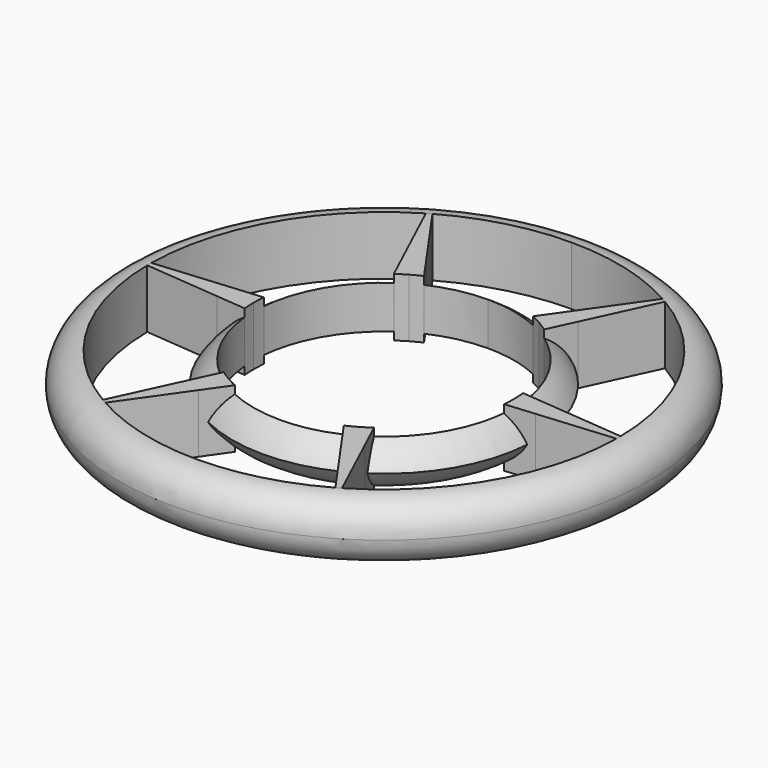
from build123d import *

# Parameters (mm, degrees)
F1_DEPTH      = 5
F3_T4_ANGLE   = 158.6510519463
F3_T9_ANGLE   = 158.6510519463
F3_T15_ANGLE  = 158.6510519463
F3_T20_ANGLE  = 158.6510519463
F3_T25_ANGLE  = 158.6510519463
F3_T31_ANGLE  = 158.6510519463
F3_T36_ANGLE  = 158.6510519463
F3_T41_ANGLE  = 158.6510519463
F3_T47_ANGLE  = 158.6510519463
F3_T52_ANGLE  = 158.6510519463
F3_T57_ANGLE  = 158.6510519463
F3_T63_ANGLE  = 158.6510519463
F3_T68_ANGLE  = 158.6510519463
F3_T73_ANGLE  = 158.6510519463
F3_T79_ANGLE  = 158.6510519463
F3_T84_ANGLE  = 158.6510519463
F3_T89_ANGLE  = 158.6510519463
F3_T95_ANGLE  = 158.6510519463
F3_T100_ANGLE = 158.6510519463
F3_T105_ANGLE = 158.6510519463
F3_T111_ANGLE = 158.6510519463
F3_T116_ANGLE = 158.6510519463
F3_T121_ANGLE = 158.6510519463
F3_T127_ANGLE = 158.6510519463
F3_T132_ANGLE = 158.6510519463
F3_T137_ANGLE = 158.6510519463
F3_T143_ANGLE = 158.6510519463
F3_T148_ANGLE = 158.6510519463
F3_T153_ANGLE = 158.6510519463
F3_T159_ANGLE = 158.6510519463
F3_T164_ANGLE = 158.6510519463
F3_T169_ANGLE = 158.6510519463
F3_T175_ANGLE = 158.6510519463
F3_T180_ANGLE = 158.6510519463
F3_T185_ANGLE = 158.6510519463
F3_T191_ANGLE = 158.6510519463


# Not quite as in the source:
# - a fillet or chamfer that OpenCascade refuses, or shapes differently, is made with other operations: its cross-section is extruded or revolved along the edge and cut away or added


with BuildPart() as f1:
    # F0 (on Top) → F1 (new body)
    with BuildSketch(Plane.XY):
        with BuildLine():
            Line((-6.4078035727, 9.0636666627), (-7.4753298331, 11.3613134754))
            ThreePointArc((-7.4753298331, 11.3613134754), (-11.7779454915, 6.8), (-13.5768510066, 0.7931687994))
            Line((-13.5768510066, 0.7931687994), (-11.0532673677, 1.0174873451))
            ThreePointArc((-11.0532673677, 1.0174873451), (-9.612881982, 5.55), (-6.4078035727, 9.0636666627))
        make_face()
        with BuildLine():
            Line((-11.0532673677, 1.0174873451), (-13.5768510066, 0.7931687994))
            ThreePointArc((-13.5768510066, 0.7931687994), (-13.5942115198, 0.3967532672), (-13.6, 0))
            Line((-13.6, 0), (-11.1, 0))
            ThreePointArc((-11.1, 0), (-11.088310687, 0.5092799909), (-11.0532673677, 1.0174873451))
        make_face()
        with BuildLine():
            ThreePointArc((-13.6, 0), (-13.5942115198, -0.3967532672), (-13.5768510066, -0.7931687994))
            Line((-13.5768510066, -0.7931687994), (-11.0532673677, -1.0174873451))
            ThreePointArc((-11.0532673677, -1.0174873451), (-11.088310687, -0.5092799909), (-11.1, 0))
            Line((-11.1, 0), (-13.6, 0))
        make_face()
        with BuildLine():
            ThreePointArc((-13.5768510066, -0.7931687994), (-11.7779454915, -6.8), (-7.4753298331, -11.3613134754))
            Line((-7.4753298331, -11.3613134754), (-6.4078035727, -9.0636666627))
            ThreePointArc((-6.4078035727, -9.0636666627), (-9.612881982, -5.55), (-11.0532673677, -1.0174873451))
            Line((-11.0532673677, -1.0174873451), (-13.5768510066, -0.7931687994))
        make_face()
        with BuildLine():
            Line((-6.4078035727, -9.0636666627), (-7.4753298331, -11.3613134754))
            ThreePointArc((-7.4753298331, -11.3613134754), (-7.1407041684, -11.5745558869), (-6.8, -11.7779454915))
            Line((-6.8, -11.7779454915), (-5.55, -9.612881982))
            ThreePointArc((-5.55, -9.612881982), (-5.9852047532, -9.3481187445), (-6.4078035727, -9.0636666627))
        make_face()
        with BuildLine():
            ThreePointArc((-6.8, -11.7779454915), (-6.4535073514, -11.9713091542), (-6.1015211735, -12.1544822748))
            Line((-6.1015211735, -12.1544822748), (-4.645463795, -10.0811540078))
            ThreePointArc((-4.645463795, -10.0811540078), (-5.1031059338, -9.8573987354), (-5.55, -9.612881982))
            Line((-5.55, -9.612881982), (-6.8, -11.7779454915))
        make_face()
        with BuildLine():
            ThreePointArc((0, -13.6), (3.135206617, -13.2336872968), (6.1015211735, -12.1544822748))
            Line((6.1015211735, -12.1544822748), (4.645463795, -10.0811540078))
            ThreePointArc((4.645463795, -10.0811540078), (2.3779392878, -10.8422970234), (0, -11.1))
            Line((0, -11.1), (0, -13.6))
        make_face()
        with BuildLine():
            Line((-4.645463795, -10.0811540078), (-6.1015211735, -12.1544822748))
            ThreePointArc((-6.1015211735, -12.1544822748), (-3.135206617, -13.2336872968), (0, -13.6))
            Line((0, -13.6), (0, -11.1))
            ThreePointArc((0, -11.1), (-2.3779392878, -10.8422970234), (-4.645463795, -10.0811540078))
        make_face()
        with BuildLine():
            Line((4.645463795, -10.0811540078), (6.1015211735, -12.1544822748))
            ThreePointArc((6.1015211735, -12.1544822748), (6.4535073514, -11.9713091542), (6.8, -11.7779454915))
            Line((6.8, -11.7779454915), (5.55, -9.612881982))
            ThreePointArc((5.55, -9.612881982), (5.1031059338, -9.8573987354), (4.645463795, -10.0811540078))
        make_face()
        with BuildLine():
            ThreePointArc((6.8, -11.7779454915), (7.1407041684, -11.5745558869), (7.4753298331, -11.3613134754))
            Line((7.4753298331, -11.3613134754), (6.4078035727, -9.0636666627))
            ThreePointArc((6.4078035727, -9.0636666627), (5.9852047532, -9.3481187445), (5.55, -9.612881982))
            Line((5.55, -9.612881982), (6.8, -11.7779454915))
        make_face()
        with BuildLine():
            ThreePointArc((7.4753298331, -11.3613134754), (11.7779454915, -6.8), (13.5768510066, -0.7931687994))
            Line((13.5768510066, -0.7931687994), (11.0532673677, -1.0174873451))
            ThreePointArc((11.0532673677, -1.0174873451), (9.612881982, -5.55), (6.4078035727, -9.0636666627))
            Line((6.4078035727, -9.0636666627), (7.4753298331, -11.3613134754))
        make_face()
        with BuildLine():
            ThreePointArc((13.5768510066, -0.7931687994), (13.5942115198, -0.3967532672), (13.6, 0))
            Line((13.6, 0), (11.1, 0))
            ThreePointArc((11.1, 0), (11.088310687, -0.5092799909), (11.0532673677, -1.0174873451))
            Line((11.0532673677, -1.0174873451), (13.5768510066, -0.7931687994))
        make_face()
        with BuildLine():
            Line((11.1, 0), (13.6, 0))
            ThreePointArc((13.6, 0), (13.5942115198, 0.3967532672), (13.5768510066, 0.7931687994))
            Line((13.5768510066, 0.7931687994), (11.0532673677, 1.0174873451))
            ThreePointArc((11.0532673677, 1.0174873451), (11.088310687, 0.5092799909), (11.1, 0))
        make_face()
        with BuildLine():
            Line((11.0532673677, 1.0174873451), (13.5768510066, 0.7931687994))
            ThreePointArc((13.5768510066, 0.7931687994), (11.7779454915, 6.8), (7.4753298331, 11.3613134754))
            Line((7.4753298331, 11.3613134754), (6.4078035727, 9.0636666627))
            ThreePointArc((6.4078035727, 9.0636666627), (9.612881982, 5.55), (11.0532673677, 1.0174873451))
        make_face()
        with BuildLine():
            Line((6.4078035727, 9.0636666627), (7.4753298331, 11.3613134754))
            ThreePointArc((7.4753298331, 11.3613134754), (7.1407041684, 11.5745558869), (6.8, 11.7779454915))
            Line((6.8, 11.7779454915), (5.55, 9.612881982))
            ThreePointArc((5.55, 9.612881982), (5.9852047532, 9.3481187445), (6.4078035727, 9.0636666627))
        make_face()
        with BuildLine():
            ThreePointArc((6.8, 11.7779454915), (6.4535073514, 11.9713091542), (6.1015211735, 12.1544822748))
            Line((6.1015211735, 12.1544822748), (4.645463795, 10.0811540078))
            ThreePointArc((4.645463795, 10.0811540078), (5.1031059338, 9.8573987354), (5.55, 9.612881982))
            Line((5.55, 9.612881982), (6.8, 11.7779454915))
        make_face()
        with BuildLine():
            Line((4.645463795, 10.0811540078), (6.1015211735, 12.1544822748))
            ThreePointArc((6.1015211735, 12.1544822748), (3.135206617, 13.2336872968), (0, 13.6))
            Line((0, 13.6), (0, 11.1))
            ThreePointArc((0, 11.1), (2.3779392878, 10.8422970234), (4.645463795, 10.0811540078))
        make_face()
        with BuildLine():
            ThreePointArc((0, 13.6), (-3.135206617, 13.2336872968), (-6.1015211735, 12.1544822748))
            Line((-6.1015211735, 12.1544822748), (-4.645463795, 10.0811540078))
            ThreePointArc((-4.645463795, 10.0811540078), (-2.3779392878, 10.8422970234), (0, 11.1))
            Line((0, 11.1), (0, 13.6))
        make_face()
        with BuildLine():
            Line((-4.645463795, 10.0811540078), (-6.1015211735, 12.1544822748))
            ThreePointArc((-6.1015211735, 12.1544822748), (-6.4535073514, 11.9713091542), (-6.8, 11.7779454915))
            Line((-6.8, 11.7779454915), (-5.55, 9.612881982))
            ThreePointArc((-5.55, 9.612881982), (-5.1031059338, 9.8573987354), (-4.645463795, 10.0811540078))
        make_face()
        with BuildLine():
            ThreePointArc((-6.8, 11.7779454915), (-7.1407041684, 11.5745558869), (-7.4753298331, 11.3613134754))
            Line((-7.4753298331, 11.3613134754), (-6.4078035727, 9.0636666627))
            ThreePointArc((-6.4078035727, 9.0636666627), (-5.9852047532, 9.3481187445), (-5.55, 9.612881982))
            Line((-5.55, 9.612881982), (-6.8, 11.7779454915))
        make_face()
        with BuildLine():
            Line((-10.1919273103, 17.2082717814), (-11.25, 19.4855715851))
            ThreePointArc((-11.25, 19.4855715851), (-19.4855715851, 11.25), (-22.5, 0))
            Line((-22.5, 0), (-19.998764173, 0.2223320735))
            ThreePointArc((-19.998764173, 0.2223320735), (-17.3205080757, 10), (-10.1919273103, 17.2082717814))
        make_face()
        with BuildLine():
            ThreePointArc((-22.5, 0), (-19.4855715851, -11.25), (-11.25, -19.4855715851))
            Line((-11.25, -19.4855715851), (-10.1919273103, -17.2082717814))
            ThreePointArc((-10.1919273103, -17.2082717814), (-17.3205080757, -10), (-19.998764173, -0.2223320735))
            Line((-19.998764173, -0.2223320735), (-22.5, 0))
        make_face()
        with BuildLine():
            ThreePointArc((-11.25, -19.4855715851), (0, -22.5), (11.25, -19.4855715851))
            Line((11.25, -19.4855715851), (9.8068368628, -17.4306038549))
            ThreePointArc((9.8068368628, -17.4306038549), (5.0689211328, -19.3469904261), (0, -20))
            ThreePointArc((0, -20), (-5.0689211328, -19.3469904261), (-9.8068368628, -17.4306038549))
            Line((-9.8068368628, -17.4306038549), (-11.25, -19.4855715851))
        make_face()
        with BuildLine():
            ThreePointArc((11.25, -19.4855715851), (19.4855715851, -11.25), (22.5, 0))
            Line((22.5, 0), (19.998764173, -0.2223320735))
            ThreePointArc((19.998764173, -0.2223320735), (17.3205080757, -10), (10.1919273103, -17.2082717814))
            Line((10.1919273103, -17.2082717814), (11.25, -19.4855715851))
        make_face()
        with BuildLine():
            Line((19.998764173, 0.2223320735), (22.5, 0))
            ThreePointArc((22.5, 0), (19.4855715851, 11.25), (11.25, 19.4855715851))
            Line((11.25, 19.4855715851), (10.1919273103, 17.2082717814))
            ThreePointArc((10.1919273103, 17.2082717814), (17.3205080757, 10), (19.998764173, 0.2223320735))
        make_face()
        with BuildLine():
            Line((9.8068368628, 17.4306038549), (11.25, 19.4855715851))
            ThreePointArc((11.25, 19.4855715851), (0, 22.5), (-11.25, 19.4855715851))
            Line((-11.25, 19.4855715851), (-9.8068368628, 17.4306038549))
            ThreePointArc((-9.8068368628, 17.4306038549), (-5.0689211328, 19.3469904261), (0, 20))
            ThreePointArc((0, 20), (5.0689211328, 19.3469904261), (9.8068368628, 17.4306038549))
        make_face()
        with BuildLine():
            Line((10.1919273103, 17.2082717814), (11.25, 19.4855715851))
            Line((11.25, 19.4855715851), (10, 17.3205080757))
            ThreePointArc((10, 17.3205080757), (10.0961196195, 17.2646566322), (10.1919273103, 17.2082717814))
        make_face()
        with BuildLine():
            Line((10, 17.3205080757), (11.25, 19.4855715851))
            Line((11.25, 19.4855715851), (9.8068368628, 17.4306038549))
            ThreePointArc((9.8068368628, 17.4306038549), (9.9035714213, 17.3758243863), (10, 17.3205080757))
        make_face()
        with BuildLine():
            Line((-9.8068368628, 17.4306038549), (-11.25, 19.4855715851))
            Line((-11.25, 19.4855715851), (-10, 17.3205080757))
            ThreePointArc((-10, 17.3205080757), (-9.9035714213, 17.3758243863), (-9.8068368628, 17.4306038549))
        make_face()
        with BuildLine():
            Line((-10, 17.3205080757), (-11.25, 19.4855715851))
            Line((-11.25, 19.4855715851), (-10.1919273103, 17.2082717814))
            ThreePointArc((-10.1919273103, 17.2082717814), (-10.0961196195, 17.2646566322), (-10, 17.3205080757))
        make_face()
        with BuildLine():
            Line((-19.998764173, 0.2223320735), (-22.5, 0))
            Line((-22.5, 0), (-20, 0))
            ThreePointArc((-20, 0), (-19.9996910409, 0.1111677541), (-19.998764173, 0.2223320735))
        make_face()
        with BuildLine():
            Line((-20, 0), (-22.5, 0))
            Line((-22.5, 0), (-19.998764173, -0.2223320735))
            ThreePointArc((-19.998764173, -0.2223320735), (-19.9996910409, -0.1111677541), (-20, 0))
        make_face()
        with BuildLine():
            Line((-10, -17.3205080757), (-11.25, -19.4855715851))
            Line((-11.25, -19.4855715851), (-9.8068368628, -17.4306038549))
            ThreePointArc((-9.8068368628, -17.4306038549), (-9.9035714213, -17.3758243863), (-10, -17.3205080757))
        make_face()
        with BuildLine():
            Line((-10.1919273103, -17.2082717814), (-11.25, -19.4855715851))
            Line((-11.25, -19.4855715851), (-10, -17.3205080757))
            ThreePointArc((-10, -17.3205080757), (-10.0961196195, -17.2646566322), (-10.1919273103, -17.2082717814))
        make_face()
        with BuildLine():
            Line((10, -17.3205080757), (11.25, -19.4855715851))
            Line((11.25, -19.4855715851), (10.1919273103, -17.2082717814))
            ThreePointArc((10.1919273103, -17.2082717814), (10.0961196195, -17.2646566322), (10, -17.3205080757))
        make_face()
        with BuildLine():
            Line((9.8068368628, -17.4306038549), (11.25, -19.4855715851))
            Line((11.25, -19.4855715851), (10, -17.3205080757))
            ThreePointArc((10, -17.3205080757), (9.9035714213, -17.3758243863), (9.8068368628, -17.4306038549))
        make_face()
        with BuildLine():
            Line((20, 0), (22.5, 0))
            Line((22.5, 0), (19.998764173, 0.2223320735))
            ThreePointArc((19.998764173, 0.2223320735), (19.9996910409, 0.1111677541), (20, 0))
        make_face()
        with BuildLine():
            Line((19.998764173, -0.2223320735), (22.5, 0))
            Line((22.5, 0), (20, 0))
            ThreePointArc((20, 0), (19.9996910409, -0.1111677541), (19.998764173, -0.2223320735))
        make_face()
        with BuildLine():
            Line((-13.5768510066, 0.7931687994), (-19.998764173, 0.2223320735))
            ThreePointArc((-19.998764173, 0.2223320735), (-19.9996910409, 0.1111677541), (-20, 0))
            Line((-20, 0), (-13.6, 0))
            ThreePointArc((-13.6, 0), (-13.5942115198, 0.3967532672), (-13.5768510066, 0.7931687994))
        make_face()
        with BuildLine():
            ThreePointArc((-20, 0), (-19.9996910409, -0.1111677541), (-19.998764173, -0.2223320735))
            Line((-19.998764173, -0.2223320735), (-13.5768510066, -0.7931687994))
            ThreePointArc((-13.5768510066, -0.7931687994), (-13.5942115198, -0.3967532672), (-13.6, 0))
            Line((-13.6, 0), (-20, 0))
        make_face()
        with BuildLine():
            Line((-6.1015211735, 12.1544822748), (-9.8068368628, 17.4306038549))
            ThreePointArc((-9.8068368628, 17.4306038549), (-9.9035714213, 17.3758243863), (-10, 17.3205080757))
            Line((-10, 17.3205080757), (-6.8, 11.7779454915))
            ThreePointArc((-6.8, 11.7779454915), (-6.4535073514, 11.9713091542), (-6.1015211735, 12.1544822748))
        make_face()
        with BuildLine():
            ThreePointArc((-10, 17.3205080757), (-10.0961196195, 17.2646566322), (-10.1919273103, 17.2082717814))
            Line((-10.1919273103, 17.2082717814), (-7.4753298331, 11.3613134754))
            ThreePointArc((-7.4753298331, 11.3613134754), (-7.1407041684, 11.5745558869), (-6.8, 11.7779454915))
            Line((-6.8, 11.7779454915), (-10, 17.3205080757))
        make_face()
        with BuildLine():
            Line((7.4753298331, 11.3613134754), (10.1919273103, 17.2082717814))
            ThreePointArc((10.1919273103, 17.2082717814), (10.0961196195, 17.2646566322), (10, 17.3205080757))
            Line((10, 17.3205080757), (6.8, 11.7779454915))
            ThreePointArc((6.8, 11.7779454915), (7.1407041684, 11.5745558869), (7.4753298331, 11.3613134754))
        make_face()
        with BuildLine():
            ThreePointArc((10, 17.3205080757), (9.9035714213, 17.3758243863), (9.8068368628, 17.4306038549))
            Line((9.8068368628, 17.4306038549), (6.1015211735, 12.1544822748))
            ThreePointArc((6.1015211735, 12.1544822748), (6.4535073514, 11.9713091542), (6.8, 11.7779454915))
            Line((6.8, 11.7779454915), (10, 17.3205080757))
        make_face()
        with BuildLine():
            ThreePointArc((19.998764173, -0.2223320735), (19.9996910409, -0.1111677541), (20, 0))
            Line((20, 0), (13.6, 0))
            ThreePointArc((13.6, 0), (13.5942115198, -0.3967532672), (13.5768510066, -0.7931687994))
            Line((13.5768510066, -0.7931687994), (19.998764173, -0.2223320735))
        make_face()
        with BuildLine():
            Line((13.6, 0), (20, 0))
            ThreePointArc((20, 0), (19.9996910409, 0.1111677541), (19.998764173, 0.2223320735))
            Line((19.998764173, 0.2223320735), (13.5768510066, 0.7931687994))
            ThreePointArc((13.5768510066, 0.7931687994), (13.5942115198, 0.3967532672), (13.6, 0))
        make_face()
        with BuildLine():
            Line((6.1015211735, -12.1544822748), (9.8068368628, -17.4306038549))
            ThreePointArc((9.8068368628, -17.4306038549), (9.9035714213, -17.3758243863), (10, -17.3205080757))
            Line((10, -17.3205080757), (6.8, -11.7779454915))
            ThreePointArc((6.8, -11.7779454915), (6.4535073514, -11.9713091542), (6.1015211735, -12.1544822748))
        make_face()
        with BuildLine():
            ThreePointArc((10, -17.3205080757), (10.0961196195, -17.2646566322), (10.1919273103, -17.2082717814))
            Line((10.1919273103, -17.2082717814), (7.4753298331, -11.3613134754))
            ThreePointArc((7.4753298331, -11.3613134754), (7.1407041684, -11.5745558869), (6.8, -11.7779454915))
            Line((6.8, -11.7779454915), (10, -17.3205080757))
        make_face()
        with BuildLine():
            Line((-7.4753298331, -11.3613134754), (-10.1919273103, -17.2082717814))
            ThreePointArc((-10.1919273103, -17.2082717814), (-10.0961196195, -17.2646566322), (-10, -17.3205080757))
            Line((-10, -17.3205080757), (-6.8, -11.7779454915))
            ThreePointArc((-6.8, -11.7779454915), (-7.1407041684, -11.5745558869), (-7.4753298331, -11.3613134754))
        make_face()
        with BuildLine():
            ThreePointArc((-10, -17.3205080757), (-9.9035714213, -17.3758243863), (-9.8068368628, -17.4306038549))
            Line((-9.8068368628, -17.4306038549), (-6.1015211735, -12.1544822748))
            ThreePointArc((-6.1015211735, -12.1544822748), (-6.4535073514, -11.9713091542), (-6.8, -11.7779454915))
            Line((-6.8, -11.7779454915), (-10, -17.3205080757))
        make_face()
    extrude(amount=-F1_DEPTH)

    # F2: fillet of radius 2.5 on 2 edges, made by hand

    # F2_s1 → F2_t2 (revolve, cut)
    with BuildSketch(Plane.XZ):
        with BuildLine():
            ThreePointArc((-22.5, -2.5), (-21.767766953, -0.732233047), (-20, 0))
            Line((-20, 0), (-22.5, 0))
            Line((-22.5, 0), (-22.5, -2.5))
        make_face()
    revolve(axis=Axis((0, 0, 0), (0, 0, 1)), mode=Mode.SUBTRACT)

    # F2_s3 → F2_t4 (revolve, cut)
    with BuildSketch(Plane.XZ):
        with BuildLine():
            ThreePointArc((-22.5, -2.5), (-21.767766953, -4.267766953), (-20, -5))
            Line((-20, -5), (-22.5, -5))
            Line((-22.5, -5), (-22.5, -2.5))
        make_face()
    revolve(axis=Axis((0, 0, -5), (0, 0, 1)), mode=Mode.SUBTRACT)

    # F3: fillet of radius 5 on 12 edges, made by hand


with BuildPart() as f3_tool2:
    # F3_s3 → F3_t4 (revolve)
    with BuildSketch(Plane(origin=(0, 0, 0), x_dir=(0, 0, 1), z_dir=(-0.9436536097, 0.3309348348, 0))):
        with BuildLine():
            ThreePointArc((0, -8.6), (-1.4644660941, -12.1355339059), (-5, -13.6))
            Line((-5, -13.6), (0, -13.6))
            Line((0, -13.6), (0, -8.6))
        make_face()
    revolve(axis=Axis((0, 0, 0), (0, 0, 1)), revolution_arc=F3_T4_ANGLE)

    split(bisect_by=Plane(origin=(-1.6302806885, -1.144913839, 0), x_dir=(0, 0, 1), z_dir=(-0.8183543157, -0.574714028, 0)), keep=Keep.TOP)


with BuildPart() as f1_1:
    add(f1.part)

    # F3_t1: cut F3_tool2
    add(f3_tool2.part, mode=Mode.SUBTRACT)


with BuildPart() as f3_tool7:
    # F3_s8 → F3_t9 (revolve)
    with BuildSketch(Plane(origin=(0, 0, 0), x_dir=(0, 0, 1), z_dir=(-0.9436536097, 0.3309348348, 0))):
        with BuildLine():
            ThreePointArc((0, -8.6), (-1.4644660941, -12.1355339059), (-5, -13.6))
            Line((-5, -13.6), (0, -13.6))
            Line((0, -13.6), (0, -8.6))
        make_face()
    revolve(axis=Axis((0, 0, 0), (0, 0, 1)), revolution_arc=F3_T9_ANGLE)

    split(bisect_by=Plane(origin=(0.1763841254, -1.9843214111, 0), x_dir=(0, 0, 1), z_dir=(0.0885397903, -0.9960726407, 0)), keep=Keep.TOP)

    split(bisect_by=Plane(origin=(1.806664814, 0.8394075721, 0), x_dir=(0, 0, 1), z_dir=(0.906894106, 0.4213586127, 0)), keep=Keep.TOP)


with BuildPart() as f1_2:
    add(f1_1.part)

    # F3_t6: cut F3_tool7
    add(f3_tool7.part, mode=Mode.SUBTRACT)


with BuildPart() as f3_tool13:
    # F3_s14 → F3_t15 (revolve)
    with BuildSketch(Plane(origin=(0, 0, 0), x_dir=(0, 0, 1), z_dir=(-0.9436536097, 0.3309348348, 0))):
        with BuildLine():
            ThreePointArc((0, -8.6), (-1.4644660941, -12.1355339059), (-5, -13.6))
            Line((-5, -13.6), (0, -13.6))
            Line((0, -13.6), (0, -8.6))
        make_face()
    revolve(axis=Axis((0, 0, 0), (0, 0, 1)), revolution_arc=F3_T15_ANGLE)

    split(bisect_by=Plane(origin=(0.1763841254, 1.9843214111, 0), x_dir=(0, 0, 1), z_dir=(0.0885397903, 0.9960726407, 0)), keep=Keep.TOP)


with BuildPart() as f1_3:
    add(f1_2.part)

    # F3_t12: cut F3_tool13
    add(f3_tool13.part, mode=Mode.SUBTRACT)


with BuildPart() as f3_tool18:
    # F3_s19 → F3_t20 (revolve)
    with BuildSketch(Plane(origin=(0, 0, 0), x_dir=(0, 0, 1), z_dir=(-0.7584247788, -0.651760581, 0))):
        with BuildLine():
            ThreePointArc((0, -8.6), (-1.4644660941, -12.1355339059), (-5, -13.6))
            Line((-5, -13.6), (0, -13.6))
            Line((0, -13.6), (0, -8.6))
        make_face()
    revolve(axis=Axis((0, 0, 0), (0, 0, 1)), revolution_arc=F3_T20_ANGLE)

    split(bisect_by=Plane(origin=(0.1763841254, -1.9843214111, 0), x_dir=(0, 0, 1), z_dir=(0.0885397903, -0.9960726407, 0)), keep=Keep.TOP)


with BuildPart() as f1_4:
    add(f1_3.part)

    # F3_t17: cut F3_tool18
    add(f3_tool18.part, mode=Mode.SUBTRACT)


with BuildPart() as f3_tool23:
    # F3_s24 → F3_t25 (revolve)
    with BuildSketch(Plane(origin=(0, 0, 0), x_dir=(0, 0, 1), z_dir=(-0.7584247788, -0.651760581, 0))):
        with BuildLine():
            ThreePointArc((0, -8.6), (-1.4644660941, -12.1355339059), (-5, -13.6))
            Line((-5, -13.6), (0, -13.6))
            Line((0, -13.6), (0, -8.6))
        make_face()
    revolve(axis=Axis((0, 0, 0), (0, 0, 1)), revolution_arc=F3_T25_ANGLE)

    split(bisect_by=Plane(origin=(1.806664814, -0.8394075721, 0), x_dir=(0, 0, 1), z_dir=(0.906894106, -0.4213586127, 0)), keep=Keep.TOP)

    split(bisect_by=Plane(origin=(0.1763841254, 1.9843214111, 0), x_dir=(0, 0, 1), z_dir=(0.0885397903, 0.9960726407, 0)), keep=Keep.TOP)


with BuildPart() as f1_5:
    add(f1_4.part)

    # F3_t22: cut F3_tool23
    add(f3_tool23.part, mode=Mode.SUBTRACT)


with BuildPart() as f3_tool29:
    # F3_s30 → F3_t31 (revolve)
    with BuildSketch(Plane(origin=(0, 0, 0), x_dir=(0, 0, 1), z_dir=(-0.7584247788, -0.651760581, 0))):
        with BuildLine():
            ThreePointArc((0, -8.6), (-1.4644660941, -12.1355339059), (-5, -13.6))
            Line((-5, -13.6), (0, -13.6))
            Line((0, -13.6), (0, -8.6))
        make_face()
    revolve(axis=Axis((0, 0, 0), (0, 0, 1)), revolution_arc=F3_T31_ANGLE)

    split(bisect_by=Plane(origin=(-1.6302806885, 1.144913839, 0), x_dir=(0, 0, 1), z_dir=(-0.8183543157, 0.574714028, 0)), keep=Keep.TOP)


with BuildPart() as f1_6:
    add(f1_5.part)

    # F3_t28: cut F3_tool29
    add(f3_tool29.part, mode=Mode.SUBTRACT)


with BuildPart() as f3_tool34:
    # F3_s35 → F3_t36 (revolve)
    with BuildSketch(Plane(origin=(0, 0, 0), x_dir=(0, 0, 1), z_dir=(0.1852288309, -0.9826954158, 0))):
        with BuildLine():
            ThreePointArc((0, -8.6), (-1.4644660941, -12.1355339059), (-5, -13.6))
            Line((-5, -13.6), (0, -13.6))
            Line((0, -13.6), (0, -8.6))
        make_face()
    revolve(axis=Axis((0, 0, 0), (0, 0, 1)), revolution_arc=F3_T36_ANGLE)

    split(bisect_by=Plane(origin=(1.806664814, -0.8394075721, 0), x_dir=(0, 0, 1), z_dir=(0.906894106, -0.4213586127, 0)), keep=Keep.TOP)


with BuildPart() as f1_7:
    add(f1_6.part)

    # F3_t33: cut F3_tool34
    add(f3_tool34.part, mode=Mode.SUBTRACT)


with BuildPart() as f3_tool39:
    # F3_s40 → F3_t41 (revolve)
    with BuildSketch(Plane(origin=(0, 0, 0), x_dir=(0, 0, 1), z_dir=(0.1852288309, -0.9826954158, 0))):
        with BuildLine():
            ThreePointArc((0, -8.6), (-1.4644660941, -12.1355339059), (-5, -13.6))
            Line((-5, -13.6), (0, -13.6))
            Line((0, -13.6), (0, -8.6))
        make_face()
    revolve(axis=Axis((0, 0, 0), (0, 0, 1)), revolution_arc=F3_T41_ANGLE)

    split(bisect_by=Plane(origin=(1.6302806885, 1.144913839, 0), x_dir=(0, 0, 1), z_dir=(0.8183543157, 0.574714028, 0)), keep=Keep.TOP)

    split(bisect_by=Plane(origin=(-1.6302806885, 1.144913839, 0), x_dir=(0, 0, 1), z_dir=(-0.8183543157, 0.574714028, 0)), keep=Keep.TOP)


with BuildPart() as f1_8:
    add(f1_7.part)

    # F3_t38: cut F3_tool39
    add(f3_tool39.part, mode=Mode.SUBTRACT)


with BuildPart() as f3_tool45:
    # F3_s46 → F3_t47 (revolve)
    with BuildSketch(Plane(origin=(0, 0, 0), x_dir=(0, 0, 1), z_dir=(0.1852288309, -0.9826954158, 0))):
        with BuildLine():
            ThreePointArc((0, -8.6), (-1.4644660941, -12.1355339059), (-5, -13.6))
            Line((-5, -13.6), (0, -13.6))
            Line((0, -13.6), (0, -8.6))
        make_face()
    revolve(axis=Axis((0, 0, 0), (0, 0, 1)), revolution_arc=F3_T47_ANGLE)

    split(bisect_by=Plane(origin=(-1.806664814, -0.8394075721, 0), x_dir=(0, 0, 1), z_dir=(-0.906894106, -0.4213586127, 0)), keep=Keep.TOP)


with BuildPart() as f1_9:
    add(f1_8.part)

    # F3_t44: cut F3_tool45
    add(f3_tool45.part, mode=Mode.SUBTRACT)


with BuildPart() as f3_tool50:
    # F3_s51 → F3_t52 (revolve)
    with BuildSketch(Plane(origin=(0, 0, 0), x_dir=(0, 0, 1), z_dir=(0.9436536097, -0.3309348348, 0))):
        with BuildLine():
            ThreePointArc((0, -8.6), (-1.4644660941, -12.1355339059), (-5, -13.6))
            Line((-5, -13.6), (0, -13.6))
            Line((0, -13.6), (0, -8.6))
        make_face()
    revolve(axis=Axis((0, 0, 0), (0, 0, 1)), revolution_arc=F3_T52_ANGLE)

    split(bisect_by=Plane(origin=(1.6302806885, 1.144913839, 0), x_dir=(0, 0, 1), z_dir=(0.8183543157, 0.574714028, 0)), keep=Keep.TOP)


with BuildPart() as f1_10:
    add(f1_9.part)

    # F3_t49: cut F3_tool50
    add(f3_tool50.part, mode=Mode.SUBTRACT)


with BuildPart() as f3_tool55:
    # F3_s56 → F3_t57 (revolve)
    with BuildSketch(Plane(origin=(0, 0, 0), x_dir=(0, 0, 1), z_dir=(0.9436536097, -0.3309348348, 0))):
        with BuildLine():
            ThreePointArc((0, -8.6), (-1.4644660941, -12.1355339059), (-5, -13.6))
            Line((-5, -13.6), (0, -13.6))
            Line((0, -13.6), (0, -8.6))
        make_face()
    revolve(axis=Axis((0, 0, 0), (0, 0, 1)), revolution_arc=F3_T57_ANGLE)

    split(bisect_by=Plane(origin=(-1.806664814, -0.8394075721, 0), x_dir=(0, 0, 1), z_dir=(-0.906894106, -0.4213586127, 0)), keep=Keep.TOP)

    split(bisect_by=Plane(origin=(-0.1763841254, 1.9843214111, 0), x_dir=(0, 0, 1), z_dir=(-0.0885397903, 0.9960726407, 0)), keep=Keep.TOP)


with BuildPart() as f1_11:
    add(f1_10.part)

    # F3_t54: cut F3_tool55
    add(f3_tool55.part, mode=Mode.SUBTRACT)


with BuildPart() as f3_tool61:
    # F3_s62 → F3_t63 (revolve)
    with BuildSketch(Plane(origin=(0, 0, 0), x_dir=(0, 0, 1), z_dir=(0.9436536097, -0.3309348348, 0))):
        with BuildLine():
            ThreePointArc((0, -8.6), (-1.4644660941, -12.1355339059), (-5, -13.6))
            Line((-5, -13.6), (0, -13.6))
            Line((0, -13.6), (0, -8.6))
        make_face()
    revolve(axis=Axis((0, 0, 0), (0, 0, 1)), revolution_arc=F3_T63_ANGLE)

    split(bisect_by=Plane(origin=(-0.1763841254, -1.9843214111, 0), x_dir=(0, 0, 1), z_dir=(-0.0885397903, -0.9960726407, 0)), keep=Keep.TOP)


with BuildPart() as f1_12:
    add(f1_11.part)

    # F3_t60: cut F3_tool61
    add(f3_tool61.part, mode=Mode.SUBTRACT)


with BuildPart() as f3_tool66:
    # F3_s67 → F3_t68 (revolve)
    with BuildSketch(Plane(origin=(0, 0, 0), x_dir=(0, 0, 1), z_dir=(0.7584247788, 0.651760581, 0))):
        with BuildLine():
            ThreePointArc((0, -8.6), (-1.4644660941, -12.1355339059), (-5, -13.6))
            Line((-5, -13.6), (0, -13.6))
            Line((0, -13.6), (0, -8.6))
        make_face()
    revolve(axis=Axis((0, 0, 0), (0, 0, 1)), revolution_arc=F3_T68_ANGLE)

    split(bisect_by=Plane(origin=(-0.1763841254, 1.9843214111, 0), x_dir=(0, 0, 1), z_dir=(-0.0885397903, 0.9960726407, 0)), keep=Keep.TOP)


with BuildPart() as f1_13:
    add(f1_12.part)

    # F3_t65: cut F3_tool66
    add(f3_tool66.part, mode=Mode.SUBTRACT)


with BuildPart() as f3_tool71:
    # F3_s72 → F3_t73 (revolve)
    with BuildSketch(Plane(origin=(0, 0, 0), x_dir=(0, 0, 1), z_dir=(0.7584247788, 0.651760581, 0))):
        with BuildLine():
            ThreePointArc((0, -8.6), (-1.4644660941, -12.1355339059), (-5, -13.6))
            Line((-5, -13.6), (0, -13.6))
            Line((0, -13.6), (0, -8.6))
        make_face()
    revolve(axis=Axis((0, 0, 0), (0, 0, 1)), revolution_arc=F3_T73_ANGLE)

    split(bisect_by=Plane(origin=(-1.806664814, 0.8394075721, 0), x_dir=(0, 0, 1), z_dir=(-0.906894106, 0.4213586127, 0)), keep=Keep.TOP)

    split(bisect_by=Plane(origin=(-0.1763841254, -1.9843214111, 0), x_dir=(0, 0, 1), z_dir=(-0.0885397903, -0.9960726407, 0)), keep=Keep.TOP)


with BuildPart() as f1_14:
    add(f1_13.part)

    # F3_t70: cut F3_tool71
    add(f3_tool71.part, mode=Mode.SUBTRACT)


with BuildPart() as f3_tool77:
    # F3_s78 → F3_t79 (revolve)
    with BuildSketch(Plane(origin=(0, 0, 0), x_dir=(0, 0, 1), z_dir=(0.7584247788, 0.651760581, 0))):
        with BuildLine():
            ThreePointArc((0, -8.6), (-1.4644660941, -12.1355339059), (-5, -13.6))
            Line((-5, -13.6), (0, -13.6))
            Line((0, -13.6), (0, -8.6))
        make_face()
    revolve(axis=Axis((0, 0, 0), (0, 0, 1)), revolution_arc=F3_T79_ANGLE)

    split(bisect_by=Plane(origin=(1.6302806885, -1.144913839, 0), x_dir=(0, 0, 1), z_dir=(0.8183543157, -0.574714028, 0)), keep=Keep.TOP)


with BuildPart() as f1_15:
    add(f1_14.part)

    # F3_t76: cut F3_tool77
    add(f3_tool77.part, mode=Mode.SUBTRACT)


with BuildPart() as f3_tool82:
    # F3_s83 → F3_t84 (revolve)
    with BuildSketch(Plane(origin=(0, 0, 0), x_dir=(0, 0, 1), z_dir=(-0.1852288309, 0.9826954158, 0))):
        with BuildLine():
            ThreePointArc((0, -8.6), (-1.4644660941, -12.1355339059), (-5, -13.6))
            Line((-5, -13.6), (0, -13.6))
            Line((0, -13.6), (0, -8.6))
        make_face()
    revolve(axis=Axis((0, 0, 0), (0, 0, 1)), revolution_arc=F3_T84_ANGLE)

    split(bisect_by=Plane(origin=(-1.806664814, 0.8394075721, 0), x_dir=(0, 0, 1), z_dir=(-0.906894106, 0.4213586127, 0)), keep=Keep.TOP)


with BuildPart() as f1_16:
    add(f1_15.part)

    # F3_t81: cut F3_tool82
    add(f3_tool82.part, mode=Mode.SUBTRACT)


with BuildPart() as f3_tool87:
    # F3_s88 → F3_t89 (revolve)
    with BuildSketch(Plane(origin=(0, 0, 0), x_dir=(0, 0, 1), z_dir=(-0.1852288309, 0.9826954158, 0))):
        with BuildLine():
            ThreePointArc((0, -8.6), (-1.4644660941, -12.1355339059), (-5, -13.6))
            Line((-5, -13.6), (0, -13.6))
            Line((0, -13.6), (0, -8.6))
        make_face()
    revolve(axis=Axis((0, 0, 0), (0, 0, 1)), revolution_arc=F3_T89_ANGLE)

    split(bisect_by=Plane(origin=(-1.6302806885, -1.144913839, 0), x_dir=(0, 0, 1), z_dir=(-0.8183543157, -0.574714028, 0)), keep=Keep.TOP)

    split(bisect_by=Plane(origin=(1.6302806885, -1.144913839, 0), x_dir=(0, 0, 1), z_dir=(0.8183543157, -0.574714028, 0)), keep=Keep.TOP)


with BuildPart() as f1_17:
    add(f1_16.part)

    # F3_t86: cut F3_tool87
    add(f3_tool87.part, mode=Mode.SUBTRACT)


with BuildPart() as f3_tool93:
    # F3_s94 → F3_t95 (revolve)
    with BuildSketch(Plane(origin=(0, 0, 0), x_dir=(0, 0, 1), z_dir=(-0.1852288309, 0.9826954158, 0))):
        with BuildLine():
            ThreePointArc((0, -8.6), (-1.4644660941, -12.1355339059), (-5, -13.6))
            Line((-5, -13.6), (0, -13.6))
            Line((0, -13.6), (0, -8.6))
        make_face()
    revolve(axis=Axis((0, 0, 0), (0, 0, 1)), revolution_arc=F3_T95_ANGLE)

    split(bisect_by=Plane(origin=(1.806664814, 0.8394075721, 0), x_dir=(0, 0, 1), z_dir=(0.906894106, 0.4213586127, 0)), keep=Keep.TOP)


with BuildPart() as f1_18:
    add(f1_17.part)

    # F3_t92: cut F3_tool93
    add(f3_tool93.part, mode=Mode.SUBTRACT)


with BuildPart() as f3_tool98:
    # F3_s99 → F3_t100 (revolve)
    with BuildSketch(Plane(origin=(0, 0, 0), x_dir=(0, 0, 1), z_dir=(0.1852288309, -0.9826954158, 0))):
        with BuildLine():
            ThreePointArc((-5, -8.6), (-3.5355339059, -12.1355339059), (0, -13.6))
            Line((0, -13.6), (-5, -13.6))
            Line((-5, -13.6), (-5, -8.6))
        make_face()
    revolve(axis=Axis((0, 0, -5), (0, 0, 1)), revolution_arc=F3_T100_ANGLE)

    split(bisect_by=Plane(origin=(1.806664814, -0.8394075721, 0), x_dir=(0, 0, 1), z_dir=(0.906894106, -0.4213586127, 0)), keep=Keep.TOP)


with BuildPart() as f1_19:
    add(f1_18.part)

    # F3_t97: cut F3_tool98
    add(f3_tool98.part, mode=Mode.SUBTRACT)


with BuildPart() as f3_tool103:
    # F3_s104 → F3_t105 (revolve)
    with BuildSketch(Plane(origin=(0, 0, 0), x_dir=(0, 0, 1), z_dir=(0.1852288309, -0.9826954158, 0))):
        with BuildLine():
            ThreePointArc((-5, -8.6), (-3.5355339059, -12.1355339059), (0, -13.6))
            Line((0, -13.6), (-5, -13.6))
            Line((-5, -13.6), (-5, -8.6))
        make_face()
    revolve(axis=Axis((0, 0, -5), (0, 0, 1)), revolution_arc=F3_T105_ANGLE)

    split(bisect_by=Plane(origin=(1.6302806885, 1.144913839, 0), x_dir=(0, 0, 1), z_dir=(0.8183543157, 0.574714028, 0)), keep=Keep.TOP)

    split(bisect_by=Plane(origin=(-1.6302806885, 1.144913839, 0), x_dir=(0, 0, 1), z_dir=(-0.8183543157, 0.574714028, 0)), keep=Keep.TOP)


with BuildPart() as f1_20:
    add(f1_19.part)

    # F3_t102: cut F3_tool103
    add(f3_tool103.part, mode=Mode.SUBTRACT)


with BuildPart() as f3_tool109:
    # F3_s110 → F3_t111 (revolve)
    with BuildSketch(Plane(origin=(0, 0, 0), x_dir=(0, 0, 1), z_dir=(0.1852288309, -0.9826954158, 0))):
        with BuildLine():
            ThreePointArc((-5, -8.6), (-3.5355339059, -12.1355339059), (0, -13.6))
            Line((0, -13.6), (-5, -13.6))
            Line((-5, -13.6), (-5, -8.6))
        make_face()
    revolve(axis=Axis((0, 0, -5), (0, 0, 1)), revolution_arc=F3_T111_ANGLE)

    split(bisect_by=Plane(origin=(-1.806664814, -0.8394075721, 0), x_dir=(0, 0, 1), z_dir=(-0.906894106, -0.4213586127, 0)), keep=Keep.TOP)


with BuildPart() as f1_21:
    add(f1_20.part)

    # F3_t108: cut F3_tool109
    add(f3_tool109.part, mode=Mode.SUBTRACT)


with BuildPart() as f3_tool114:
    # F3_s115 → F3_t116 (revolve)
    with BuildSketch(Plane(origin=(0, 0, 0), x_dir=(0, 0, 1), z_dir=(-0.7584247788, -0.651760581, 0))):
        with BuildLine():
            ThreePointArc((-5, -8.6), (-3.5355339059, -12.1355339059), (0, -13.6))
            Line((0, -13.6), (-5, -13.6))
            Line((-5, -13.6), (-5, -8.6))
        make_face()
    revolve(axis=Axis((0, 0, -5), (0, 0, 1)), revolution_arc=F3_T116_ANGLE)

    split(bisect_by=Plane(origin=(0.1763841254, -1.9843214111, 0), x_dir=(0, 0, 1), z_dir=(0.0885397903, -0.9960726407, 0)), keep=Keep.TOP)


with BuildPart() as f1_22:
    add(f1_21.part)

    # F3_t113: cut F3_tool114
    add(f3_tool114.part, mode=Mode.SUBTRACT)


with BuildPart() as f3_tool119:
    # F3_s120 → F3_t121 (revolve)
    with BuildSketch(Plane(origin=(0, 0, 0), x_dir=(0, 0, 1), z_dir=(-0.7584247788, -0.651760581, 0))):
        with BuildLine():
            ThreePointArc((-5, -8.6), (-3.5355339059, -12.1355339059), (0, -13.6))
            Line((0, -13.6), (-5, -13.6))
            Line((-5, -13.6), (-5, -8.6))
        make_face()
    revolve(axis=Axis((0, 0, -5), (0, 0, 1)), revolution_arc=F3_T121_ANGLE)

    split(bisect_by=Plane(origin=(1.806664814, -0.8394075721, 0), x_dir=(0, 0, 1), z_dir=(0.906894106, -0.4213586127, 0)), keep=Keep.TOP)

    split(bisect_by=Plane(origin=(0.1763841254, 1.9843214111, 0), x_dir=(0, 0, 1), z_dir=(0.0885397903, 0.9960726407, 0)), keep=Keep.TOP)


with BuildPart() as f1_23:
    add(f1_22.part)

    # F3_t118: cut F3_tool119
    add(f3_tool119.part, mode=Mode.SUBTRACT)


with BuildPart() as f3_tool125:
    # F3_s126 → F3_t127 (revolve)
    with BuildSketch(Plane(origin=(0, 0, 0), x_dir=(0, 0, 1), z_dir=(-0.7584247788, -0.651760581, 0))):
        with BuildLine():
            ThreePointArc((-5, -8.6), (-3.5355339059, -12.1355339059), (0, -13.6))
            Line((0, -13.6), (-5, -13.6))
            Line((-5, -13.6), (-5, -8.6))
        make_face()
    revolve(axis=Axis((0, 0, -5), (0, 0, 1)), revolution_arc=F3_T127_ANGLE)

    split(bisect_by=Plane(origin=(-1.6302806885, 1.144913839, 0), x_dir=(0, 0, 1), z_dir=(-0.8183543157, 0.574714028, 0)), keep=Keep.TOP)


with BuildPart() as f1_24:
    add(f1_23.part)

    # F3_t124: cut F3_tool125
    add(f3_tool125.part, mode=Mode.SUBTRACT)


with BuildPart() as f3_tool130:
    # F3_s131 → F3_t132 (revolve)
    with BuildSketch(Plane(origin=(0, 0, 0), x_dir=(0, 0, 1), z_dir=(0.9436536097, -0.3309348348, 0))):
        with BuildLine():
            ThreePointArc((-5, -8.6), (-3.5355339059, -12.1355339059), (0, -13.6))
            Line((0, -13.6), (-5, -13.6))
            Line((-5, -13.6), (-5, -8.6))
        make_face()
    revolve(axis=Axis((0, 0, -5), (0, 0, 1)), revolution_arc=F3_T132_ANGLE)

    split(bisect_by=Plane(origin=(1.6302806885, 1.144913839, 0), x_dir=(0, 0, 1), z_dir=(0.8183543157, 0.574714028, 0)), keep=Keep.TOP)


with BuildPart() as f1_25:
    add(f1_24.part)

    # F3_t129: cut F3_tool130
    add(f3_tool130.part, mode=Mode.SUBTRACT)


with BuildPart() as f3_tool135:
    # F3_s136 → F3_t137 (revolve)
    with BuildSketch(Plane(origin=(0, 0, 0), x_dir=(0, 0, 1), z_dir=(0.9436536097, -0.3309348348, 0))):
        with BuildLine():
            ThreePointArc((-5, -8.6), (-3.5355339059, -12.1355339059), (0, -13.6))
            Line((0, -13.6), (-5, -13.6))
            Line((-5, -13.6), (-5, -8.6))
        make_face()
    revolve(axis=Axis((0, 0, -5), (0, 0, 1)), revolution_arc=F3_T137_ANGLE)

    split(bisect_by=Plane(origin=(-1.806664814, -0.8394075721, 0), x_dir=(0, 0, 1), z_dir=(-0.906894106, -0.4213586127, 0)), keep=Keep.TOP)

    split(bisect_by=Plane(origin=(-0.1763841254, 1.9843214111, 0), x_dir=(0, 0, 1), z_dir=(-0.0885397903, 0.9960726407, 0)), keep=Keep.TOP)


with BuildPart() as f1_26:
    add(f1_25.part)

    # F3_t134: cut F3_tool135
    add(f3_tool135.part, mode=Mode.SUBTRACT)


with BuildPart() as f3_tool141:
    # F3_s142 → F3_t143 (revolve)
    with BuildSketch(Plane(origin=(0, 0, 0), x_dir=(0, 0, 1), z_dir=(0.9436536097, -0.3309348348, 0))):
        with BuildLine():
            ThreePointArc((-5, -8.6), (-3.5355339059, -12.1355339059), (0, -13.6))
            Line((0, -13.6), (-5, -13.6))
            Line((-5, -13.6), (-5, -8.6))
        make_face()
    revolve(axis=Axis((0, 0, -5), (0, 0, 1)), revolution_arc=F3_T143_ANGLE)

    split(bisect_by=Plane(origin=(-0.1763841254, -1.9843214111, 0), x_dir=(0, 0, 1), z_dir=(-0.0885397903, -0.9960726407, 0)), keep=Keep.TOP)


with BuildPart() as f1_27:
    add(f1_26.part)

    # F3_t140: cut F3_tool141
    add(f3_tool141.part, mode=Mode.SUBTRACT)


with BuildPart() as f3_tool146:
    # F3_s147 → F3_t148 (revolve)
    with BuildSketch(Plane(origin=(0, 0, 0), x_dir=(0, 0, 1), z_dir=(0.7584247788, 0.651760581, 0))):
        with BuildLine():
            ThreePointArc((-5, -8.6), (-3.5355339059, -12.1355339059), (0, -13.6))
            Line((0, -13.6), (-5, -13.6))
            Line((-5, -13.6), (-5, -8.6))
        make_face()
    revolve(axis=Axis((0, 0, -5), (0, 0, 1)), revolution_arc=F3_T148_ANGLE)

    split(bisect_by=Plane(origin=(-0.1763841254, 1.9843214111, 0), x_dir=(0, 0, 1), z_dir=(-0.0885397903, 0.9960726407, 0)), keep=Keep.TOP)


with BuildPart() as f1_28:
    add(f1_27.part)

    # F3_t145: cut F3_tool146
    add(f3_tool146.part, mode=Mode.SUBTRACT)


with BuildPart() as f3_tool151:
    # F3_s152 → F3_t153 (revolve)
    with BuildSketch(Plane(origin=(0, 0, 0), x_dir=(0, 0, 1), z_dir=(0.7584247788, 0.651760581, 0))):
        with BuildLine():
            ThreePointArc((-5, -8.6), (-3.5355339059, -12.1355339059), (0, -13.6))
            Line((0, -13.6), (-5, -13.6))
            Line((-5, -13.6), (-5, -8.6))
        make_face()
    revolve(axis=Axis((0, 0, -5), (0, 0, 1)), revolution_arc=F3_T153_ANGLE)

    split(bisect_by=Plane(origin=(-1.806664814, 0.8394075721, 0), x_dir=(0, 0, 1), z_dir=(-0.906894106, 0.4213586127, 0)), keep=Keep.TOP)

    split(bisect_by=Plane(origin=(-0.1763841254, -1.9843214111, 0), x_dir=(0, 0, 1), z_dir=(-0.0885397903, -0.9960726407, 0)), keep=Keep.TOP)


with BuildPart() as f1_29:
    add(f1_28.part)

    # F3_t150: cut F3_tool151
    add(f3_tool151.part, mode=Mode.SUBTRACT)


with BuildPart() as f3_tool157:
    # F3_s158 → F3_t159 (revolve)
    with BuildSketch(Plane(origin=(0, 0, 0), x_dir=(0, 0, 1), z_dir=(0.7584247788, 0.651760581, 0))):
        with BuildLine():
            ThreePointArc((-5, -8.6), (-3.5355339059, -12.1355339059), (0, -13.6))
            Line((0, -13.6), (-5, -13.6))
            Line((-5, -13.6), (-5, -8.6))
        make_face()
    revolve(axis=Axis((0, 0, -5), (0, 0, 1)), revolution_arc=F3_T159_ANGLE)

    split(bisect_by=Plane(origin=(1.6302806885, -1.144913839, 0), x_dir=(0, 0, 1), z_dir=(0.8183543157, -0.574714028, 0)), keep=Keep.TOP)


with BuildPart() as f1_30:
    add(f1_29.part)

    # F3_t156: cut F3_tool157
    add(f3_tool157.part, mode=Mode.SUBTRACT)


with BuildPart() as f3_tool162:
    # F3_s163 → F3_t164 (revolve)
    with BuildSketch(Plane(origin=(0, 0, 0), x_dir=(0, 0, 1), z_dir=(-0.1852288309, 0.9826954158, 0))):
        with BuildLine():
            ThreePointArc((-5, -8.6), (-3.5355339059, -12.1355339059), (0, -13.6))
            Line((0, -13.6), (-5, -13.6))
            Line((-5, -13.6), (-5, -8.6))
        make_face()
    revolve(axis=Axis((0, 0, -5), (0, 0, 1)), revolution_arc=F3_T164_ANGLE)

    split(bisect_by=Plane(origin=(-1.806664814, 0.8394075721, 0), x_dir=(0, 0, 1), z_dir=(-0.906894106, 0.4213586127, 0)), keep=Keep.TOP)


with BuildPart() as f1_31:
    add(f1_30.part)

    # F3_t161: cut F3_tool162
    add(f3_tool162.part, mode=Mode.SUBTRACT)


with BuildPart() as f3_tool167:
    # F3_s168 → F3_t169 (revolve)
    with BuildSketch(Plane(origin=(0, 0, 0), x_dir=(0, 0, 1), z_dir=(-0.1852288309, 0.9826954158, 0))):
        with BuildLine():
            ThreePointArc((-5, -8.6), (-3.5355339059, -12.1355339059), (0, -13.6))
            Line((0, -13.6), (-5, -13.6))
            Line((-5, -13.6), (-5, -8.6))
        make_face()
    revolve(axis=Axis((0, 0, -5), (0, 0, 1)), revolution_arc=F3_T169_ANGLE)

    split(bisect_by=Plane(origin=(-1.6302806885, -1.144913839, 0), x_dir=(0, 0, 1), z_dir=(-0.8183543157, -0.574714028, 0)), keep=Keep.TOP)

    split(bisect_by=Plane(origin=(1.6302806885, -1.144913839, 0), x_dir=(0, 0, 1), z_dir=(0.8183543157, -0.574714028, 0)), keep=Keep.TOP)


with BuildPart() as f1_32:
    add(f1_31.part)

    # F3_t166: cut F3_tool167
    add(f3_tool167.part, mode=Mode.SUBTRACT)


with BuildPart() as f3_tool173:
    # F3_s174 → F3_t175 (revolve)
    with BuildSketch(Plane(origin=(0, 0, 0), x_dir=(0, 0, 1), z_dir=(-0.1852288309, 0.9826954158, 0))):
        with BuildLine():
            ThreePointArc((-5, -8.6), (-3.5355339059, -12.1355339059), (0, -13.6))
            Line((0, -13.6), (-5, -13.6))
            Line((-5, -13.6), (-5, -8.6))
        make_face()
    revolve(axis=Axis((0, 0, -5), (0, 0, 1)), revolution_arc=F3_T175_ANGLE)

    split(bisect_by=Plane(origin=(1.806664814, 0.8394075721, 0), x_dir=(0, 0, 1), z_dir=(0.906894106, 0.4213586127, 0)), keep=Keep.TOP)


with BuildPart() as f1_33:
    add(f1_32.part)

    # F3_t172: cut F3_tool173
    add(f3_tool173.part, mode=Mode.SUBTRACT)


with BuildPart() as f3_tool178:
    # F3_s179 → F3_t180 (revolve)
    with BuildSketch(Plane(origin=(0, 0, 0), x_dir=(0, 0, 1), z_dir=(-0.9436536097, 0.3309348348, 0))):
        with BuildLine():
            ThreePointArc((-5, -8.6), (-3.5355339059, -12.1355339059), (0, -13.6))
            Line((0, -13.6), (-5, -13.6))
            Line((-5, -13.6), (-5, -8.6))
        make_face()
    revolve(axis=Axis((0, 0, -5), (0, 0, 1)), revolution_arc=F3_T180_ANGLE)

    split(bisect_by=Plane(origin=(-1.6302806885, -1.144913839, 0), x_dir=(0, 0, 1), z_dir=(-0.8183543157, -0.574714028, 0)), keep=Keep.TOP)


with BuildPart() as f1_34:
    add(f1_33.part)

    # F3_t177: cut F3_tool178
    add(f3_tool178.part, mode=Mode.SUBTRACT)


with BuildPart() as f3_tool183:
    # F3_s184 → F3_t185 (revolve)
    with BuildSketch(Plane(origin=(0, 0, 0), x_dir=(0, 0, 1), z_dir=(-0.9436536097, 0.3309348348, 0))):
        with BuildLine():
            ThreePointArc((-5, -8.6), (-3.5355339059, -12.1355339059), (0, -13.6))
            Line((0, -13.6), (-5, -13.6))
            Line((-5, -13.6), (-5, -8.6))
        make_face()
    revolve(axis=Axis((0, 0, -5), (0, 0, 1)), revolution_arc=F3_T185_ANGLE)

    split(bisect_by=Plane(origin=(0.1763841254, -1.9843214111, 0), x_dir=(0, 0, 1), z_dir=(0.0885397903, -0.9960726407, 0)), keep=Keep.TOP)

    split(bisect_by=Plane(origin=(1.806664814, 0.8394075721, 0), x_dir=(0, 0, 1), z_dir=(0.906894106, 0.4213586127, 0)), keep=Keep.TOP)


with BuildPart() as f1_35:
    add(f1_34.part)

    # F3_t182: cut F3_tool183
    add(f3_tool183.part, mode=Mode.SUBTRACT)


with BuildPart() as f3_tool189:
    # F3_s190 → F3_t191 (revolve)
    with BuildSketch(Plane(origin=(0, 0, 0), x_dir=(0, 0, 1), z_dir=(-0.9436536097, 0.3309348348, 0))):
        with BuildLine():
            ThreePointArc((-5, -8.6), (-3.5355339059, -12.1355339059), (0, -13.6))
            Line((0, -13.6), (-5, -13.6))
            Line((-5, -13.6), (-5, -8.6))
        make_face()
    revolve(axis=Axis((0, 0, -5), (0, 0, 1)), revolution_arc=F3_T191_ANGLE)

    split(bisect_by=Plane(origin=(0.1763841254, 1.9843214111, 0), x_dir=(0, 0, 1), z_dir=(0.0885397903, 0.9960726407, 0)), keep=Keep.TOP)


with BuildPart() as f1_36:
    add(f1_35.part)

    # F3_t188: cut F3_tool189
    add(f3_tool189.part, mode=Mode.SUBTRACT)


solid = f1_36.part
